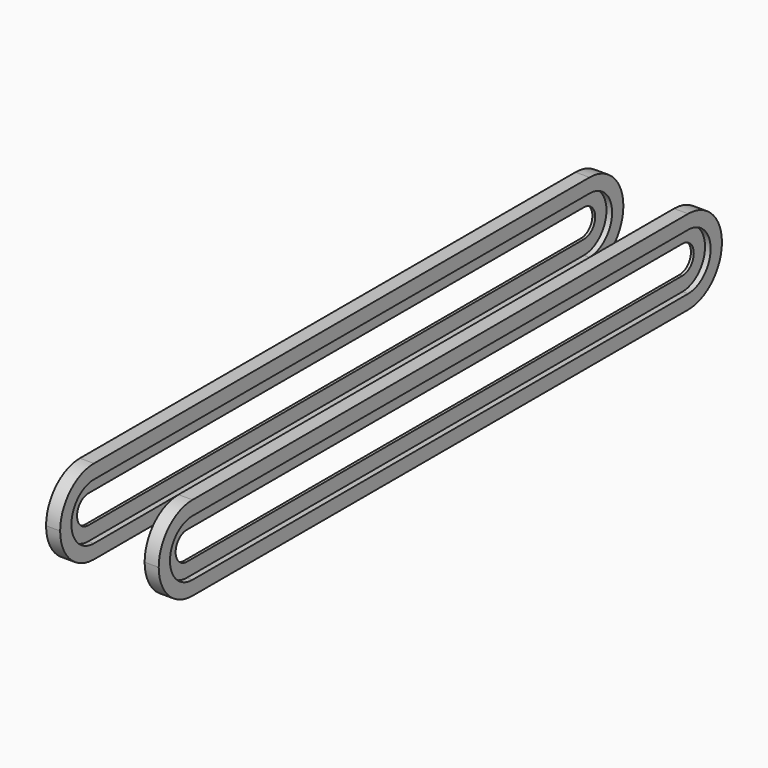
from build123d import *

# Parameters (mm, degrees)
F1_DEPTH      = 125
F1_DEPTH_BACK = 125
F6_DEPTH      = 5.001
F7_DEPTH      = 5.001
F8_DEPTH      = 2
F9_DEPTH      = 2
F10_DEPTH     = 2
F11_DEPTH     = 2
F12_W         = 30
F12_H         = 250
F13_DEPTH     = 30.001
F14_R         = 14.99999


# Not quite as in the source:
# - a fillet or chamfer is up to 0.001 mm smaller than in the source, because OpenCascade refuses the exact size


with BuildPart() as f1:
    # F0 (on Front) → F1 (new body, two sides)
    with BuildSketch(Plane.XZ) as f1_sk:
        Polygon((20, -15), (20, 15), (-20, 15), (-20, -15), (-15, -15), (-15, 10), (15, 10), (15, -15), align=None)
    extrude(amount=F1_DEPTH)
    extrude(f1_sk.sketch, amount=-F1_DEPTH_BACK)

    # F2 (on face) → F6 (cut, through all)
    with BuildSketch(Plane(origin=(15, 0, 0), x_dir=(0, -1, 0), z_dir=(-1, 0, 0))):
        with BuildLine():
            Line((-110, -5), (110, -5))
            ThreePointArc((110, -5), (115, 0), (110, 5))
            Line((110, 5), (-110, 5))
            ThreePointArc((-110, 5), (-115, 0), (-110, -5))
        make_face()
    extrude(amount=-F6_DEPTH, mode=Mode.SUBTRACT)

    # F4 (on face) → F7 (cut, through all)
    with BuildSketch(Plane.YZ.offset(-15)):
        with BuildLine():
            Line((110, 5), (-110, 5))
            ThreePointArc((-110, 5), (-115, 0), (-110, -5))
            Line((-110, -5), (110, -5))
            ThreePointArc((110, -5), (115, 0), (110, 5))
        make_face()
    extrude(amount=-F7_DEPTH, mode=Mode.SUBTRACT)

    # F2 (on face) → F8 (cut)
    with BuildSketch(Plane(origin=(15, 0, 0), x_dir=(0, -1, 0), z_dir=(-1, 0, 0))):
        with BuildLine():
            Line((-110, -10), (110, -10))
            ThreePointArc((110, -10), (120, 0), (110, 10))
            Line((110, 10), (-110, 10))
            ThreePointArc((-110, 10), (-120, 0), (-110, -10))
        make_face()
        with BuildLine():
            ThreePointArc((110, 5), (115, 0), (110, -5))
            Line((110, -5), (-110, -5))
            ThreePointArc((-110, -5), (-115, 0), (-110, 5))
            Line((-110, 5), (110, 5))
        make_face(mode=Mode.SUBTRACT)
    extrude(amount=-F8_DEPTH, mode=Mode.SUBTRACT)

    # F3 (on face) → F9 (cut)
    with BuildSketch(Plane.YZ.offset(20)):
        with BuildLine():
            ThreePointArc((-110, 10), (-120, 0), (-110, -10))
            Line((-110, -10), (110, -10))
            ThreePointArc((110, -10), (120, 0), (110, 10))
            Line((110, 10), (-110, 10))
        make_face()
        with BuildLine():
            ThreePointArc((-110, -5), (-115, 0), (-110, 5))
            Line((-110, 5), (110, 5))
            ThreePointArc((110, 5), (115, 0), (110, -5))
            Line((110, -5), (-110, -5))
        make_face(mode=Mode.SUBTRACT)
    extrude(amount=-F9_DEPTH, mode=Mode.SUBTRACT)

    # F5 (on face) → F10 (cut)
    with BuildSketch(Plane(origin=(-20, 0, 0), x_dir=(0, -1, 0), z_dir=(-1, 0, 0))):
        with BuildLine():
            Line((110, 10), (-110, 10))
            ThreePointArc((-110, 10), (-120, 0), (-110, -10))
            Line((-110, -10), (110, -10))
            ThreePointArc((110, -10), (120, 0), (110, 10))
        make_face()
        with BuildLine():
            ThreePointArc((-110, -5), (-115, 0), (-110, 5))
            Line((-110, 5), (110, 5))
            ThreePointArc((110, 5), (115, 0), (110, -5))
            Line((110, -5), (-110, -5))
        make_face(mode=Mode.SUBTRACT)
    extrude(amount=-F10_DEPTH, mode=Mode.SUBTRACT)

    # F4 (on face) → F11 (cut)
    with BuildSketch(Plane.YZ.offset(-15)):
        with BuildLine():
            Line((110, 10), (-110, 10))
            ThreePointArc((-110, 10), (-120, 0), (-110, -10))
            Line((-110, -10), (110, -10))
            ThreePointArc((110, -10), (120, 0), (110, 10))
        make_face()
        with BuildLine():
            ThreePointArc((-110, -5), (-115, 0), (-110, 5))
            Line((-110, 5), (110, 5))
            ThreePointArc((110, 5), (115, 0), (110, -5))
            Line((110, -5), (-110, -5))
        make_face(mode=Mode.SUBTRACT)
    extrude(amount=-F11_DEPTH, mode=Mode.SUBTRACT)

    # F12 (on face) → F13 (cut, through all)
    with BuildSketch(Plane.XY.offset(15)):
        Rectangle(F12_W, F12_H)
    extrude(amount=-F13_DEPTH, mode=Mode.SUBTRACT)

    # F14 (radius 15 in the source; OpenCascade refuses exactly that, so slightly less here)
    f14_edges = [f1.edges().sort_by_distance(p)[0] for p in [
        (-17.5, 125, -15),
        (17.5, 125, -15),
        (-17.5, -125, -15),
        (17.5, -125, -15),
        (-17.5, 125, 15),
        (17.5, 125, 15),
        (-17.5, -125, 15),
        (17.5, -125, 15),
    ]]
    fillet(f14_edges, radius=F14_R)


solid = f1.part
